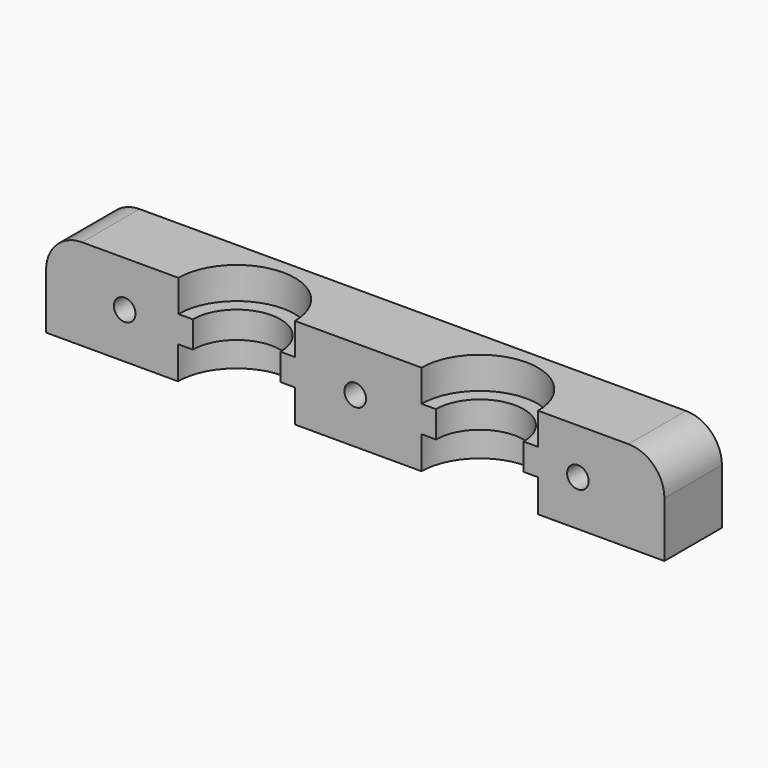
from build123d import *

# Parameters (mm, degrees)
F0_W     = 86
F0_H     = 10
F1_DEPTH = 12.69
F2_W     = 6.1
F2_H     = 3.7164622918
F4_W     = 6.1
F4_H     = 3.7164622918
F6_R     = 5
F7_R     = 1.5
F8_DEPTH = 10.001


# Not quite as in the source:
# - a feature names something its author has since deleted; it is built from what else it names


with BuildPart() as f1:
    # F0 (on Top) → F1 (new body)
    with BuildSketch(Plane.XY):
        Rectangle(F0_W, F0_H)
    extrude(amount=F1_DEPTH)

    # F2 (on face) → F3 (revolve, cut)
    with BuildSketch(Plane.XZ.offset(5)):
        Polygon((-8.4, 12.69), (-16.5, 12.69), (-16.5, 8.2610268146), (-10.4, 8.2610268146), (-8.4, 8.2610268146), align=None)
        with Locations((-13.45, 6.4027956687)):
            Rectangle(F2_W, F2_H)
        Polygon((-10.4, 4.5445645228), (-16.5, 4.5445645228), (-16.5, 0), (-8.3565199748, 0), (-8.3565199748, 4.5445645228), align=None)
    revolve(axis=Axis((-16.5, -5, 6.345), (0, 0, -1)), mode=Mode.SUBTRACT)

    # F4 (on face) → F5 (revolve, cut)
    with BuildSketch(Plane.XZ.offset(5)):
        Polygon((25.4217400126, 12.69), (17.3217400126, 12.69), (17.3217400126, 8.2610268146), (23.4217400126, 8.2610268146), (25.4217400126, 8.2610268146), align=None)
        with Locations((20.3717400126, 6.4027956687)):
            Rectangle(F4_W, F4_H)
        Polygon((23.4217400126, 4.5445645228), (17.3217400126, 4.5445645228), (17.3217400126, 0), (25.4217400126, 0), (25.4217400126, 4.5445645228), align=None)
    revolve(axis=Axis((17.3217400126, -5, 6.345), (0, 0, -1)), mode=Mode.SUBTRACT)

    # F6
    f6_edges = [f1.edges().sort_by_distance(p)[0] for p in [
        (-43, 0, 12.69),
        (43, 0, 12.69),
    ]]
    fillet(f6_edges, radius=F6_R)

    # F7 (on face) → F8 (cut, through all)
    with BuildSketch(Plane(origin=(0, 5, 0), x_dir=(-1, 0, 0), z_dir=(0, 1, 0))):
        with Locations((-30.9640802443, 6.345)):
            Circle(F7_R)
        with Locations((0, 6.345)):
            Circle(F7_R)
        with Locations((32.0656448603, 6.345)):
            Circle(F7_R)
    extrude(amount=-F8_DEPTH, mode=Mode.SUBTRACT)


solid = f1.part
